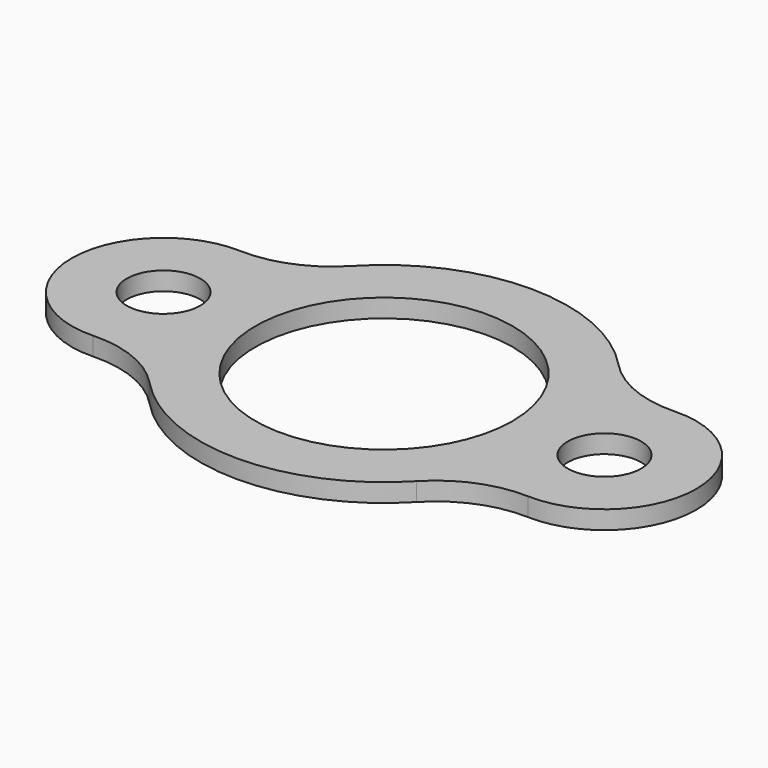
from build123d import *

# Parameters (mm, degrees)
F0_R     = 12.7
F0_R_2   = 44.45
F1_DEPTH = 6.35
F2_DEPTH = 254


# Not quite as in the source:
# - an extrude ends at something that could not be found from the text; its depth is read off the source's solid


with BuildPart() as f1:
    # F0 (on Top) → F1 (new body)
    with BuildSketch(Plane.XY):
        with BuildLine():
            ThreePointArc((75.1176136364, 31.7315448688), (59.3475236203, 34.5646316236), (46.13671875, 43.6308741946))
            ThreePointArc((46.13671875, 43.6308741946), (0, 63.5), (-46.13671875, 43.6308741946))
            ThreePointArc((-46.13671875, 43.6308741946), (-59.3475236203, 34.5646316236), (-75.1176136364, 31.7315448688))
            ThreePointArc((-75.1176136364, 31.7315448688), (-107.95, 0), (-75.1176136364, -31.7315448688))
            ThreePointArc((-75.1176136364, -31.7315448688), (-59.3475236203, -34.5646316236), (-46.13671875, -43.6308741946))
            ThreePointArc((-46.13671875, -43.6308741946), (0, -63.5), (46.13671875, -43.6308741946))
            ThreePointArc((46.13671875, -43.6308741946), (59.3475236203, -34.5646316236), (75.1176136364, -31.7315448688))
            ThreePointArc((75.1176136364, -31.7315448688), (107.95, 0), (75.1176136364, 31.7315448688))
        make_face()
        with Locations((-76.2, 0)):
            Circle(F0_R, mode=Mode.SUBTRACT)
        Circle(F0_R_2, mode=Mode.SUBTRACT)
        with Locations((76.2, 0)):
            Circle(F0_R, mode=Mode.SUBTRACT)
    extrude(amount=F1_DEPTH)

    # F0 (on Top) → F2 (cut, through all)
    with BuildSketch(Plane.XY):
        Circle(F0_R_2)
    extrude(amount=-F2_DEPTH, mode=Mode.SUBTRACT)


solid = f1.part
